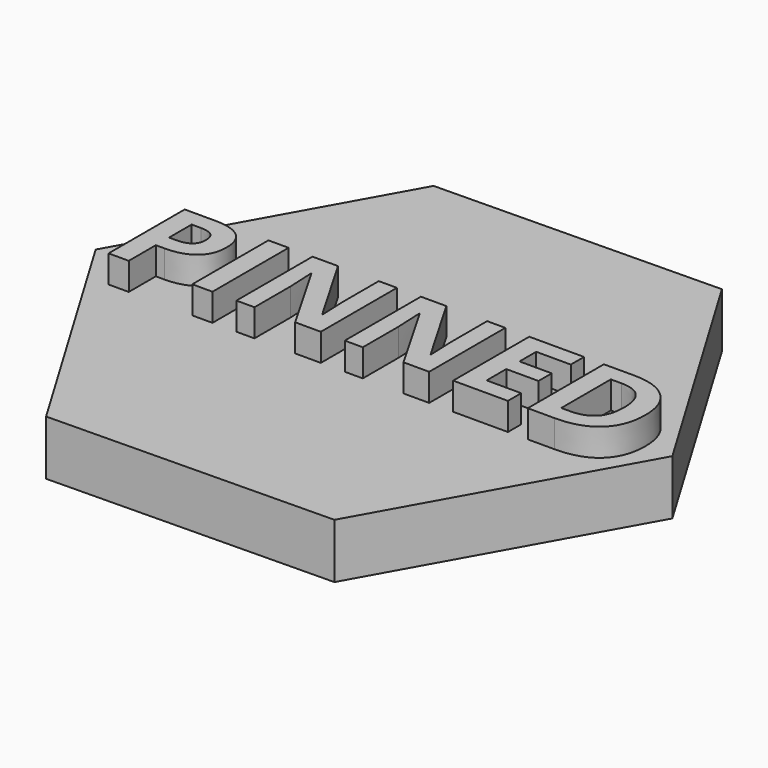
from build123d import *

# Parameters (mm, degrees)
F1_DEPTH     = 2
F2_TEXT_SIZE = 4.8611111111
F3_DEPTH     = 1


# Not quite as in the source:
# - Text() gives the source's letters only with a copy of the font that has no kerning and outlines rounded to 1/6400 em; it was checked with that copy


with BuildPart() as f1:
    # F0 (on Top) → F1 (new body)
    with BuildSketch(Plane.XY):
        Polygon((-15.9115251625, 22.8344005057), (-10.8492016447, 31.91166666), (-16.1791829723, 40.8344005057), (-26.5714878177, 40.6798681972), (-31.6338113355, 31.6026020429), (-26.3038300079, 22.6798681972), align=None)
    extrude(amount=F1_DEPTH)

    # F2 (on face) → F3 (join)
    with BuildSketch(Plane.XY.offset(2)):
        with Locations((-30.4366852254, 30.148806722)):
            Text('PINNED', F2_TEXT_SIZE, font='Open Sans', font_style=FontStyle.BOLD, text_align=(TextAlign.LEFT, TextAlign.BOTTOM))
    extrude(amount=F3_DEPTH)


solid = f1.part
